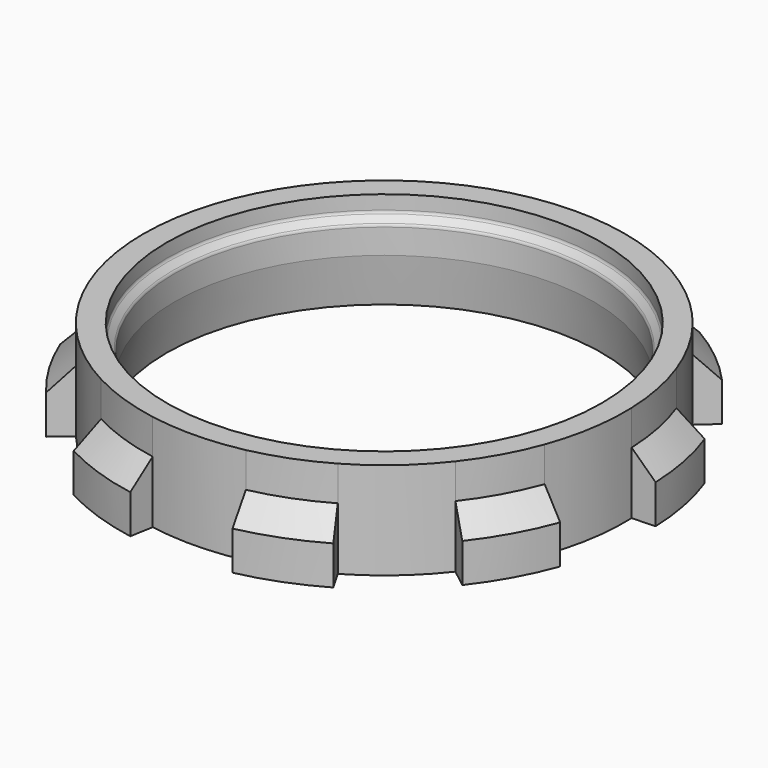
from build123d import *

# Parameters (mm, degrees)
F3_DEPTH        = 25.4
F3_COPIES_COUNT = 9


# Not quite as in the source:
# - a pattern or mirror of a feature is missing from the dataset's text; its kind, count and spacing are read off the source's solid


with BuildPart() as f1:
    # F0 (on Front) → F1 (revolve)
    with BuildSketch(Plane.XZ):
        with BuildLine():
            Line((-43.18, 15.875), (-43.18, 0))
            Line((-43.18, 0), (-35.56, 0))
            Line((-35.56, 0), (-34.29, 7.747))
            Line((-34.29, 7.747), (-34.29, 11.8019743879))
            ThreePointArc((-34.29, 11.8019743879), (-34.3383364969, 12.0449783674), (-34.4759871939, 12.2509871939))
            Line((-34.4759871939, 12.2509871939), (-35.3740128061, 13.1490128061))
            ThreePointArc((-35.3740128061, 13.1490128061), (-35.5116635031, 13.3550216326), (-35.56, 13.5980256121))
            Line((-35.56, 13.5980256121), (-35.56, 15.875))
            Line((-35.56, 15.875), (-43.18, 15.875))
        make_face()
    revolve(axis=Axis((0, 0, 20.137766609), (0, 0, 1)))

    # F2 (on face) → F3 (cut)
    with BuildSketch(Plane(origin=(0, 0, 0), x_dir=(1, 0, 0), z_dir=(0, 0, -1))):
        with BuildLine():
            Line((-49.9110633764, 0), (-39.37, 0))
            ThreePointArc((-39.37, 0), (-38.6466622123, 7.512150148), (-36.5032283543, 14.7482615828))
            Line((-36.5032283543, 14.7482615828), (-46.2767321268, 18.6970134252))
            ThreePointArc((-46.2767321268, 18.6970134252), (-48.994056565, 9.523479861), (-49.9110633764, 0))
        make_face()
    f3 = extrude(amount=-F3_DEPTH, mode=Mode.SUBTRACT)

    # F3_copies: F3 ×9 about axis
    f3_copies_axis = Axis((0, 0, 0), (0, 0, 1))
    for i in range(1, F3_COPIES_COUNT):
        add(f3.rotate(f3_copies_axis, i * 360 / F3_COPIES_COUNT), mode=Mode.SUBTRACT)

    # F5 (on Right) → F6 (revolve, cut)
    with BuildSketch(Plane.YZ):
        Polygon((39.37, 15.875), (39.37, 10.16), (43.18, 6.35), (43.18, 15.875), align=None)
    revolve(axis=Axis((0, 0, 20.137766609), (0, 0, 1)), mode=Mode.SUBTRACT)


solid = f1.part
